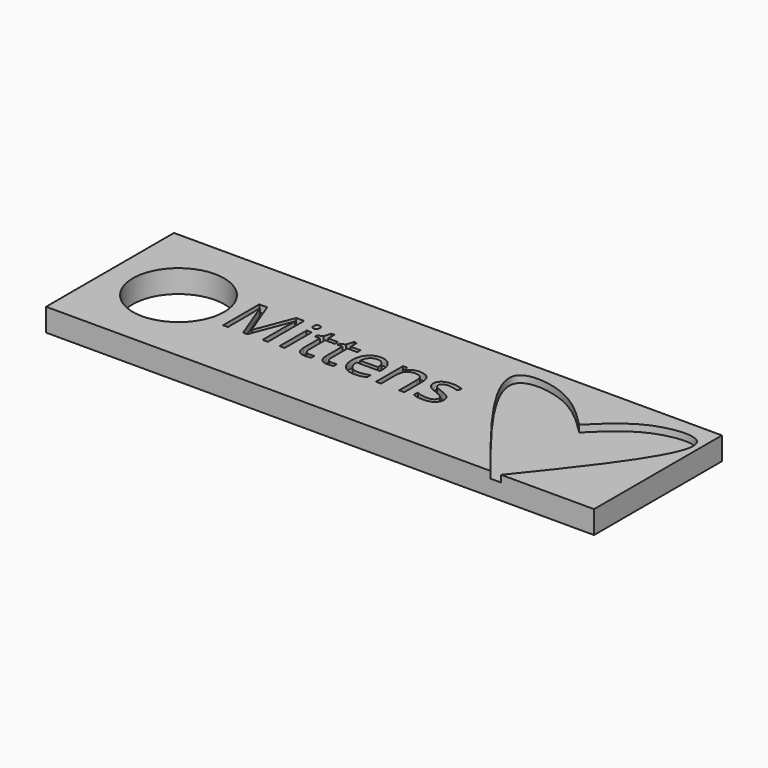
from build123d import *

# Parameters (mm, degrees)
F0_W         = 120
F0_H         = 35
F0_R         = 10
F1_DEPTH     = 5
F2_TEXT_SIZE = 13.8888888889
F4_DEPTH     = 1.5
F5_DEPTH     = 1.5
F6_DEPTH     = 1.5


# Not quite as in the source:
# - Text() gives the source's letters only with a copy of the font that has no kerning and outlines rounded to 1/6400 em; it was checked with that copy


with BuildPart() as f1:
    # F0 (on Top) → F1 (new body)
    with BuildSketch(Plane.XY):
        Rectangle(F0_W, F0_H)
        with Locations((-45, 0)):
            Circle(F0_R, mode=Mode.SUBTRACT)
    extrude(amount=F1_DEPTH)

    # F2 (on face) → F4 (cut)
    with BuildSketch(Plane.XY.offset(5)):
        with Locations((-33.4485928437, -3.9534885337)):
            Text('Mittens', F2_TEXT_SIZE, font='Open Sans', text_align=(TextAlign.LEFT, TextAlign.BOTTOM))
    extrude(amount=F4_DEPTH, mode=Mode.SUBTRACT)

    # F3 (on face) → F5 (cut)
    with BuildSketch(Plane.XY.offset(5)):
        with BuildLine():
            add(Edge.make_bspline(
                [(38.4868457913, 5.3289476782), (41.5209217249, 8.359982491), (47.1549283062, 13.9883419841), (66.2751837918, 15.5515252753), (49.586266239, -5.1675700787), (38.4868457913, -18.9473703504)],
                knots=[0, 0, 0, 0, 0.2810148028, 0.5218192568, 1, 1, 1, 1], degree=3))
            add(Edge.make_bspline(
                [(38.4868457913, 5.3289476782), (35.4527698578, 8.359982491), (29.8187632765, 13.9883419841), (10.6985077909, 15.5515252753), (27.3874253437, -5.1675700787), (38.4868457913, -18.9473703504)],
                knots=[0, 0, 0, 0, 0.2810148028, 0.5218192568, 1, 1, 1, 1], degree=3))
        make_face()
    extrude(amount=-F5_DEPTH, mode=Mode.SUBTRACT)

    # F2 (on face) → F6 (cut)
    with BuildSketch(Plane.XY.offset(5)):
        with Locations((-33.4485928437, -3.9534885337)):
            Text('Mittens', F2_TEXT_SIZE, font='Open Sans', text_align=(TextAlign.LEFT, TextAlign.BOTTOM))
    extrude(amount=-F6_DEPTH, mode=Mode.SUBTRACT)


solid = f1.part
